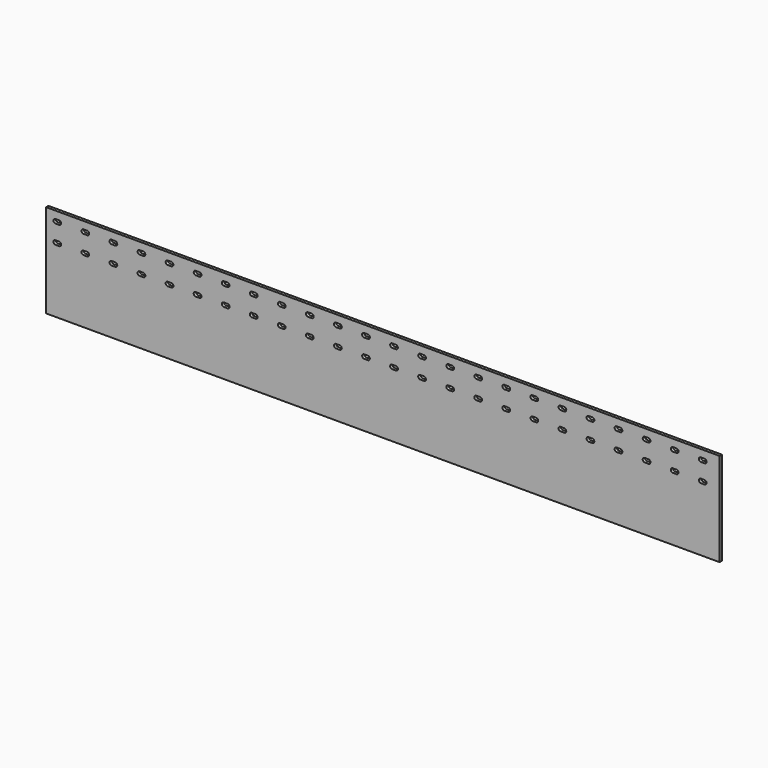
from build123d import *

# Parameters (mm, degrees)
F0_W          = 1828.8
F0_H          = 254
F1_DEPTH      = 3.96875
F1_DEPTH_BACK = 3.96875
F3_DEPTH      = 7.9375


# Not quite as in the source:
# - a length typed as a fraction of an inch, garbled in the dataset ("3 / 203.2 mm" for 3/8 in), is restored


with BuildPart() as f1:
    # F0 (on Front) → F1 (new body, two sides)
    with BuildSketch(Plane.XZ) as f1_sk:
        with Locations((914.4, 127)):
            Rectangle(F0_W, F0_H)
    extrude(amount=F1_DEPTH)
    extrude(f1_sk.sketch, amount=-F1_DEPTH_BACK)

    # F2 (on face) → F3 (cut, through all)
    with BuildSketch(Plane.XZ.offset(3.96875)):
        with BuildLine():
            Line((35.4, 234.1), (25.4, 234.1))
            ThreePointArc((25.4, 234.1), (19.9, 228.6), (25.4, 223.1))
            Line((25.4, 223.1), (35.4, 223.1))
            ThreePointArc((35.4, 223.1), (40.9, 228.6), (35.4, 234.1))
        make_face()
        with BuildLine():
            Line((101.6, 223.1), (111.6, 223.1))
            ThreePointArc((111.6, 223.1), (117.1, 228.6), (111.6, 234.1))
            Line((111.6, 234.1), (101.6, 234.1))
            ThreePointArc((101.6, 234.1), (96.1, 228.6), (101.6, 223.1))
        make_face()
        with BuildLine():
            Line((101.6, 172.3), (111.6, 172.3))
            ThreePointArc((111.6, 172.3), (117.1, 177.8), (111.6, 183.3))
            Line((111.6, 183.3), (101.6, 183.3))
            ThreePointArc((101.6, 183.3), (96.1, 177.8), (101.6, 172.3))
        make_face()
        with BuildLine():
            Line((25.4, 172.3), (35.4, 172.3))
            ThreePointArc((35.4, 172.3), (40.9, 177.8), (35.4, 183.3))
            Line((35.4, 183.3), (25.4, 183.3))
            ThreePointArc((25.4, 183.3), (19.9, 177.8), (25.4, 172.3))
        make_face()
        with BuildLine():
            Line((177.8, 223.1), (187.8, 223.1))
            ThreePointArc((187.8, 223.1), (193.3, 228.6), (187.8, 234.1))
            Line((187.8, 234.1), (177.8, 234.1))
            ThreePointArc((177.8, 234.1), (172.3, 228.6), (177.8, 223.1))
        make_face()
        with BuildLine():
            Line((177.8, 172.3), (187.8, 172.3))
            ThreePointArc((187.8, 172.3), (193.3, 177.8), (187.8, 183.3))
            Line((187.8, 183.3), (177.8, 183.3))
            ThreePointArc((177.8, 183.3), (172.3, 177.8), (177.8, 172.3))
        make_face()
        with BuildLine():
            Line((254, 223.1), (264, 223.1))
            ThreePointArc((264, 223.1), (269.5, 228.6), (264, 234.1))
            Line((264, 234.1), (254, 234.1))
            ThreePointArc((254, 234.1), (248.5, 228.6), (254, 223.1))
        make_face()
        with BuildLine():
            Line((254, 172.3), (264, 172.3))
            ThreePointArc((264, 172.3), (269.5, 177.8), (264, 183.3))
            Line((264, 183.3), (254, 183.3))
            ThreePointArc((254, 183.3), (248.5, 177.8), (254, 172.3))
        make_face()
        with BuildLine():
            Line((330.2, 172.3), (340.2, 172.3))
            ThreePointArc((340.2, 172.3), (345.7, 177.8), (340.2, 183.3))
            Line((340.2, 183.3), (330.2, 183.3))
            ThreePointArc((330.2, 183.3), (324.7, 177.8), (330.2, 172.3))
        make_face()
        with BuildLine():
            Line((330.2, 223.1), (340.2, 223.1))
            ThreePointArc((340.2, 223.1), (345.7, 228.6), (340.2, 234.1))
            Line((340.2, 234.1), (330.2, 234.1))
            ThreePointArc((330.2, 234.1), (324.7, 228.6), (330.2, 223.1))
        make_face()
        with BuildLine():
            Line((406.4, 223.1), (416.4, 223.1))
            ThreePointArc((416.4, 223.1), (421.9, 228.6), (416.4, 234.1))
            Line((416.4, 234.1), (406.4, 234.1))
            ThreePointArc((406.4, 234.1), (400.9, 228.6), (406.4, 223.1))
        make_face()
        with BuildLine():
            Line((406.4, 172.3), (416.4, 172.3))
            ThreePointArc((416.4, 172.3), (421.9, 177.8), (416.4, 183.3))
            Line((416.4, 183.3), (406.4, 183.3))
            ThreePointArc((406.4, 183.3), (400.9, 177.8), (406.4, 172.3))
        make_face()
        with BuildLine():
            Line((482.6, 172.3), (492.6, 172.3))
            ThreePointArc((492.6, 172.3), (498.1, 177.8), (492.6, 183.3))
            Line((492.6, 183.3), (482.6, 183.3))
            ThreePointArc((482.6, 183.3), (477.1, 177.8), (482.6, 172.3))
        make_face()
        with BuildLine():
            Line((482.6, 223.1), (492.6, 223.1))
            ThreePointArc((492.6, 223.1), (498.1, 228.6), (492.6, 234.1))
            Line((492.6, 234.1), (482.6, 234.1))
            ThreePointArc((482.6, 234.1), (477.1, 228.6), (482.6, 223.1))
        make_face()
        with BuildLine():
            Line((558.8, 223.1), (568.8, 223.1))
            ThreePointArc((568.8, 223.1), (574.3, 228.6), (568.8, 234.1))
            Line((568.8, 234.1), (558.8, 234.1))
            ThreePointArc((558.8, 234.1), (553.3, 228.6), (558.8, 223.1))
        make_face()
        with BuildLine():
            Line((558.8, 172.3), (568.8, 172.3))
            ThreePointArc((568.8, 172.3), (574.3, 177.8), (568.8, 183.3))
            Line((568.8, 183.3), (558.8, 183.3))
            ThreePointArc((558.8, 183.3), (553.3, 177.8), (558.8, 172.3))
        make_face()
        with BuildLine():
            Line((635, 223.1), (645, 223.1))
            ThreePointArc((645, 223.1), (650.5, 228.6), (645, 234.1))
            Line((645, 234.1), (635, 234.1))
            ThreePointArc((635, 234.1), (629.5, 228.6), (635, 223.1))
        make_face()
        with BuildLine():
            Line((635, 172.3), (645, 172.3))
            ThreePointArc((645, 172.3), (650.5, 177.8), (645, 183.3))
            Line((645, 183.3), (635, 183.3))
            ThreePointArc((635, 183.3), (629.5, 177.8), (635, 172.3))
        make_face()
        with BuildLine():
            Line((711.2, 223.1), (721.2, 223.1))
            ThreePointArc((721.2, 223.1), (726.7, 228.6), (721.2, 234.1))
            Line((721.2, 234.1), (711.2, 234.1))
            ThreePointArc((711.2, 234.1), (705.7, 228.6), (711.2, 223.1))
        make_face()
        with BuildLine():
            Line((787.4, 172.3), (797.4, 172.3))
            ThreePointArc((797.4, 172.3), (802.9, 177.8), (797.4, 183.3))
            Line((797.4, 183.3), (787.4, 183.3))
            ThreePointArc((787.4, 183.3), (781.9, 177.8), (787.4, 172.3))
        make_face()
        with BuildLine():
            Line((787.4, 223.1), (797.4, 223.1))
            ThreePointArc((797.4, 223.1), (802.9, 228.6), (797.4, 234.1))
            Line((797.4, 234.1), (787.4, 234.1))
            ThreePointArc((787.4, 234.1), (781.9, 228.6), (787.4, 223.1))
        make_face()
        with BuildLine():
            Line((711.2, 172.3), (721.2, 172.3))
            ThreePointArc((721.2, 172.3), (726.7, 177.8), (721.2, 183.3))
            Line((721.2, 183.3), (711.2, 183.3))
            ThreePointArc((711.2, 183.3), (705.7, 177.8), (711.2, 172.3))
        make_face()
        with BuildLine():
            Line((863.6, 223.1), (873.6, 223.1))
            ThreePointArc((873.6, 223.1), (879.1, 228.6), (873.6, 234.1))
            Line((873.6, 234.1), (863.6, 234.1))
            ThreePointArc((863.6, 234.1), (858.1, 228.6), (863.6, 223.1))
        make_face()
        with BuildLine():
            Line((863.6, 172.3), (873.6, 172.3))
            ThreePointArc((873.6, 172.3), (879.1, 177.8), (873.6, 183.3))
            Line((873.6, 183.3), (863.6, 183.3))
            ThreePointArc((863.6, 183.3), (858.1, 177.8), (863.6, 172.3))
        make_face()
        with BuildLine():
            Line((939.8, 172.3), (949.8, 172.3))
            ThreePointArc((949.8, 172.3), (955.3, 177.8), (949.8, 183.3))
            Line((949.8, 183.3), (939.8, 183.3))
            ThreePointArc((939.8, 183.3), (934.3, 177.8), (939.8, 172.3))
        make_face()
        with BuildLine():
            Line((939.8, 223.1), (949.8, 223.1))
            ThreePointArc((949.8, 223.1), (955.3, 228.6), (949.8, 234.1))
            Line((949.8, 234.1), (939.8, 234.1))
            ThreePointArc((939.8, 234.1), (934.3, 228.6), (939.8, 223.1))
        make_face()
        with BuildLine():
            Line((1016, 223.1), (1026, 223.1))
            ThreePointArc((1026, 223.1), (1031.5, 228.6), (1026, 234.1))
            Line((1026, 234.1), (1016, 234.1))
            ThreePointArc((1016, 234.1), (1010.5, 228.6), (1016, 223.1))
        make_face()
        with BuildLine():
            Line((1016, 172.3), (1026, 172.3))
            ThreePointArc((1026, 172.3), (1031.5, 177.8), (1026, 183.3))
            Line((1026, 183.3), (1016, 183.3))
            ThreePointArc((1016, 183.3), (1010.5, 177.8), (1016, 172.3))
        make_face()
        with BuildLine():
            Line((1092.2, 172.3), (1102.2, 172.3))
            ThreePointArc((1102.2, 172.3), (1107.7, 177.8), (1102.2, 183.3))
            Line((1102.2, 183.3), (1092.2, 183.3))
            ThreePointArc((1092.2, 183.3), (1086.7, 177.8), (1092.2, 172.3))
        make_face()
        with BuildLine():
            Line((1092.2, 223.1), (1102.2, 223.1))
            ThreePointArc((1102.2, 223.1), (1107.7, 228.6), (1102.2, 234.1))
            Line((1102.2, 234.1), (1092.2, 234.1))
            ThreePointArc((1092.2, 234.1), (1086.7, 228.6), (1092.2, 223.1))
        make_face()
        with BuildLine():
            Line((1168.4, 223.1), (1178.4, 223.1))
            ThreePointArc((1178.4, 223.1), (1183.9, 228.6), (1178.4, 234.1))
            Line((1178.4, 234.1), (1168.4, 234.1))
            ThreePointArc((1168.4, 234.1), (1162.9, 228.6), (1168.4, 223.1))
        make_face()
        with BuildLine():
            Line((1168.4, 172.3), (1178.4, 172.3))
            ThreePointArc((1178.4, 172.3), (1183.9, 177.8), (1178.4, 183.3))
            Line((1178.4, 183.3), (1168.4, 183.3))
            ThreePointArc((1168.4, 183.3), (1162.9, 177.8), (1168.4, 172.3))
        make_face()
        with BuildLine():
            Line((1244.6, 172.3), (1254.6, 172.3))
            ThreePointArc((1254.6, 172.3), (1260.1, 177.8), (1254.6, 183.3))
            Line((1254.6, 183.3), (1244.6, 183.3))
            ThreePointArc((1244.6, 183.3), (1239.1, 177.8), (1244.6, 172.3))
        make_face()
        with BuildLine():
            Line((1244.6, 223.1), (1254.6, 223.1))
            ThreePointArc((1254.6, 223.1), (1260.1, 228.6), (1254.6, 234.1))
            Line((1254.6, 234.1), (1244.6, 234.1))
            ThreePointArc((1244.6, 234.1), (1239.1, 228.6), (1244.6, 223.1))
        make_face()
        with BuildLine():
            Line((1320.8, 223.1), (1330.8, 223.1))
            ThreePointArc((1330.8, 223.1), (1336.3, 228.6), (1330.8, 234.1))
            Line((1330.8, 234.1), (1320.8, 234.1))
            ThreePointArc((1320.8, 234.1), (1315.3, 228.6), (1320.8, 223.1))
        make_face()
        with BuildLine():
            Line((1320.8, 172.3), (1330.8, 172.3))
            ThreePointArc((1330.8, 172.3), (1336.3, 177.8), (1330.8, 183.3))
            Line((1330.8, 183.3), (1320.8, 183.3))
            ThreePointArc((1320.8, 183.3), (1315.3, 177.8), (1320.8, 172.3))
        make_face()
        with BuildLine():
            Line((1397, 172.3), (1407, 172.3))
            ThreePointArc((1407, 172.3), (1412.5, 177.8), (1407, 183.3))
            Line((1407, 183.3), (1397, 183.3))
            ThreePointArc((1397, 183.3), (1391.5, 177.8), (1397, 172.3))
        make_face()
        with BuildLine():
            Line((1397, 223.1), (1407, 223.1))
            ThreePointArc((1407, 223.1), (1412.5, 228.6), (1407, 234.1))
            Line((1407, 234.1), (1397, 234.1))
            ThreePointArc((1397, 234.1), (1391.5, 228.6), (1397, 223.1))
        make_face()
        with BuildLine():
            Line((1473.2, 223.1), (1483.2, 223.1))
            ThreePointArc((1483.2, 223.1), (1488.7, 228.6), (1483.2, 234.1))
            Line((1483.2, 234.1), (1473.2, 234.1))
            ThreePointArc((1473.2, 234.1), (1467.7, 228.6), (1473.2, 223.1))
        make_face()
        with BuildLine():
            Line((1473.2, 172.3), (1483.2, 172.3))
            ThreePointArc((1483.2, 172.3), (1488.7, 177.8), (1483.2, 183.3))
            Line((1483.2, 183.3), (1473.2, 183.3))
            ThreePointArc((1473.2, 183.3), (1467.7, 177.8), (1473.2, 172.3))
        make_face()
        with BuildLine():
            Line((1549.4, 172.3), (1559.4, 172.3))
            ThreePointArc((1559.4, 172.3), (1564.9, 177.8), (1559.4, 183.3))
            Line((1559.4, 183.3), (1549.4, 183.3))
            ThreePointArc((1549.4, 183.3), (1543.9, 177.8), (1549.4, 172.3))
        make_face()
        with BuildLine():
            Line((1549.4, 223.1), (1559.4, 223.1))
            ThreePointArc((1559.4, 223.1), (1564.9, 228.6), (1559.4, 234.1))
            Line((1559.4, 234.1), (1549.4, 234.1))
            ThreePointArc((1549.4, 234.1), (1543.9, 228.6), (1549.4, 223.1))
        make_face()
        with BuildLine():
            Line((1625.6, 223.1), (1635.6, 223.1))
            ThreePointArc((1635.6, 223.1), (1641.1, 228.6), (1635.6, 234.1))
            Line((1635.6, 234.1), (1625.6, 234.1))
            ThreePointArc((1625.6, 234.1), (1620.1, 228.6), (1625.6, 223.1))
        make_face()
        with BuildLine():
            Line((1625.6, 172.3), (1635.6, 172.3))
            ThreePointArc((1635.6, 172.3), (1641.1, 177.8), (1635.6, 183.3))
            Line((1635.6, 183.3), (1625.6, 183.3))
            ThreePointArc((1625.6, 183.3), (1620.1, 177.8), (1625.6, 172.3))
        make_face()
        with BuildLine():
            Line((1701.8, 172.3), (1711.8, 172.3))
            ThreePointArc((1711.8, 172.3), (1717.3, 177.8), (1711.8, 183.3))
            Line((1711.8, 183.3), (1701.8, 183.3))
            ThreePointArc((1701.8, 183.3), (1696.3, 177.8), (1701.8, 172.3))
        make_face()
        with BuildLine():
            Line((1701.8, 223.1), (1711.8, 223.1))
            ThreePointArc((1711.8, 223.1), (1717.3, 228.6), (1711.8, 234.1))
            Line((1711.8, 234.1), (1701.8, 234.1))
            ThreePointArc((1701.8, 234.1), (1696.3, 228.6), (1701.8, 223.1))
        make_face()
        with BuildLine():
            Line((1778, 223.1), (1788, 223.1))
            ThreePointArc((1788, 223.1), (1793.5, 228.6), (1788, 234.1))
            Line((1788, 234.1), (1778, 234.1))
            ThreePointArc((1778, 234.1), (1772.5, 228.6), (1778, 223.1))
        make_face()
        with BuildLine():
            Line((1778, 172.3), (1788, 172.3))
            ThreePointArc((1788, 172.3), (1793.5, 177.8), (1788, 183.3))
            Line((1788, 183.3), (1778, 183.3))
            ThreePointArc((1778, 183.3), (1772.5, 177.8), (1778, 172.3))
        make_face()
    extrude(amount=-F3_DEPTH, mode=Mode.SUBTRACT)


solid = f1.part
